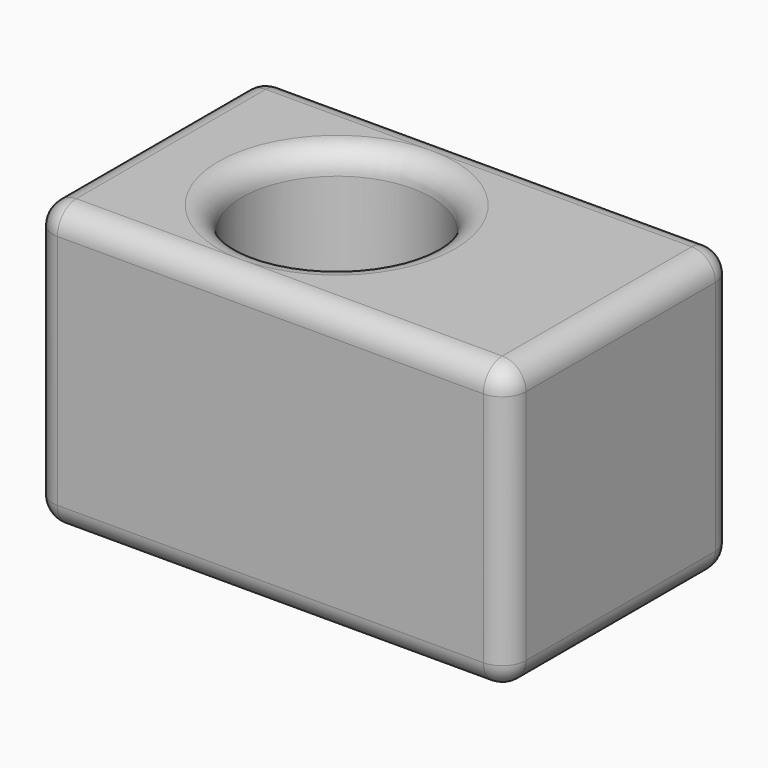
from build123d import *

# Parameters (mm, degrees)
F0_W     = 101.6
F0_H     = 76.2
F0_R     = 25.4
F1_DEPTH = 38.1
F2_DEPTH = 25.4
F3_R     = 6.34999


# Not quite as in the source:
# - a fillet or chamfer is up to 0.001 mm smaller than in the source, because OpenCascade refuses the exact size


with BuildPart() as f1:
    # F0 (on Top) → F1 (new body, symmetric)
    with BuildSketch(Plane.XY):
        Rectangle(F0_W, F0_H)
        Circle(F0_R, mode=Mode.SUBTRACT)
    extrude(amount=F1_DEPTH, both=True)

    # F2 (add): a face of the model
    f2_faces = [f1.faces().sort_by_distance(p)[0] for p in [
        (50.8, 0, 0),
    ]]
    extrude(f2_faces, amount=F2_DEPTH)

    # F3 (radius 6.35 in the source; OpenCascade refuses exactly that, so slightly less here)
    f3_edges = [f1.edges().sort_by_distance(p)[0] for p in [
        (12.7, 38.1, 38.1),
        (-50.8, 0, 38.1),
        (12.7, -38.1, 38.1),
        (76.2, 0, 38.1),
        (-25.4, 0, 38.1),
        (-50.8, 38.1, 0),
        (-50.8, 0, -38.1),
        (-50.8, -38.1, 0),
        (76.2, 38.1, 0),
        (12.7, 38.1, -38.1),
        (12.7, -38.1, -38.1),
        (76.2, -38.1, 0),
        (76.2, 0, -38.1),
        (-25.4, 0, -38.1),
    ]]
    fillet(f3_edges, radius=F3_R)


solid = f1.part
